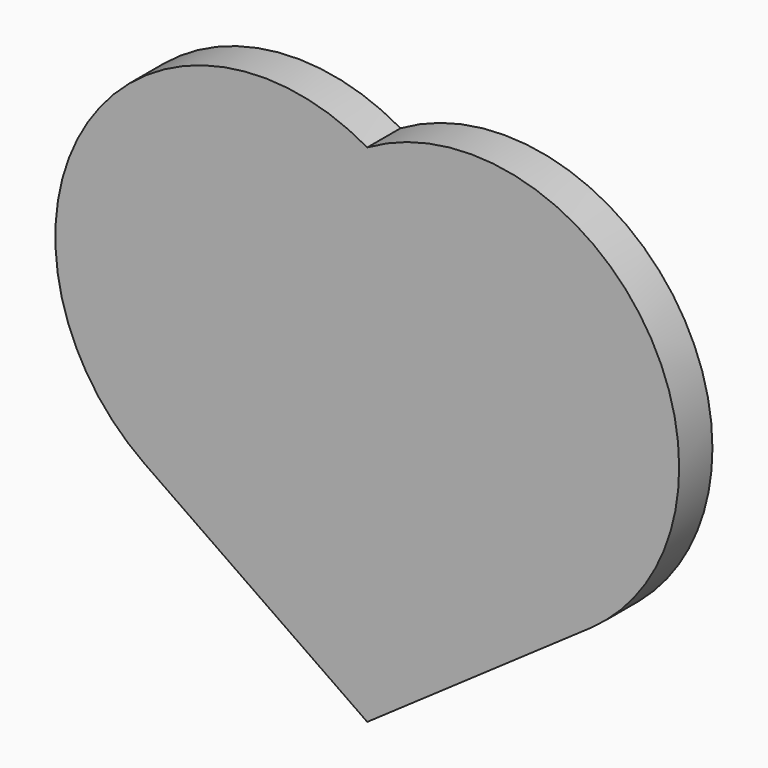
from build123d import *

# Parameters (mm, degrees)
F1_DEPTH = 2.54
F2_DEPTH = 5.08


# Not quite as in the source:
# - a feature names something its author has since deleted; it is built from what else it names


with BuildPart() as f1:
    # F0 (on Front) → F1 (new body)
    with BuildSketch(Plane.XZ):
        with BuildLine():
            ThreePointArc((25.4, 0), (21.9970452561, -12.7), (12.7, -21.9970452561))
            ThreePointArc((12.7, -21.9970452561), (26.4693193728, -25.3774812793), (39.9054559874, -20.8507013455))
            ThreePointArc((39.9054559874, -20.8507013455), (47.9122031583, -11.762682898), (50.8, 0))
            ThreePointArc((50.8, 0), (38.1, 21.9970452561), (12.7, 21.9970452561))
            ThreePointArc((12.7, 21.9970452561), (21.9970452561, 12.7), (25.4, 0))
        make_face()
        with BuildLine():
            ThreePointArc((12.7, 21.9970452561), (0, 0), (12.7, -21.9970452561))
            ThreePointArc((12.7, -21.9970452561), (21.9970452561, -12.7), (25.4, 0))
            ThreePointArc((25.4, 0), (21.9970452561, 12.7), (12.7, 21.9970452561))
        make_face()
    extrude(amount=F1_DEPTH)

    # F0 (on Front) → F2 (join)
    with BuildSketch(Plane.XZ):
        with BuildLine():
            ThreePointArc((12.7, 21.9970452561), (-21.4428837855, 13.6147983812), (-14.5054559874, -20.8507013455))
            ThreePointArc((-14.5054559874, -20.8507013455), (-1.0693193728, -25.3774812793), (12.7, -21.9970452561))
            ThreePointArc((12.7, -21.9970452561), (0, 0), (12.7, 21.9970452561))
        make_face()
        with BuildLine():
            ThreePointArc((12.7, -21.9970452561), (-1.0693193728, -25.3774812793), (-14.5054559874, -20.8507013455))
            Line((-14.5054559874, -20.8507013455), (12.7, -39.7770452561))
            Line((12.7, -39.7770452561), (12.7, -21.9970452561))
        make_face()
        with BuildLine():
            ThreePointArc((12.7, 21.9970452561), (0, 0), (12.7, -21.9970452561))
            ThreePointArc((12.7, -21.9970452561), (21.9970452561, -12.7), (25.4, 0))
            ThreePointArc((25.4, 0), (21.9970452561, 12.7), (12.7, 21.9970452561))
        make_face()
        with BuildLine():
            ThreePointArc((25.4, 0), (21.9970452561, -12.7), (12.7, -21.9970452561))
            ThreePointArc((12.7, -21.9970452561), (26.4693193728, -25.3774812793), (39.9054559874, -20.8507013455))
            ThreePointArc((39.9054559874, -20.8507013455), (47.9122031583, -11.762682898), (50.8, 0))
            ThreePointArc((50.8, 0), (38.1, 21.9970452561), (12.7, 21.9970452561))
            ThreePointArc((12.7, 21.9970452561), (21.9970452561, 12.7), (25.4, 0))
        make_face()
        with BuildLine():
            ThreePointArc((39.9054559874, -20.8507013455), (26.4693193728, -25.3774812793), (12.7, -21.9970452561))
            Line((12.7, -21.9970452561), (12.7, -39.7770452561))
            Line((12.7, -39.7770452561), (39.9054559874, -20.8507013455))
        make_face()
    extrude(amount=F2_DEPTH)


solid = f1.part
